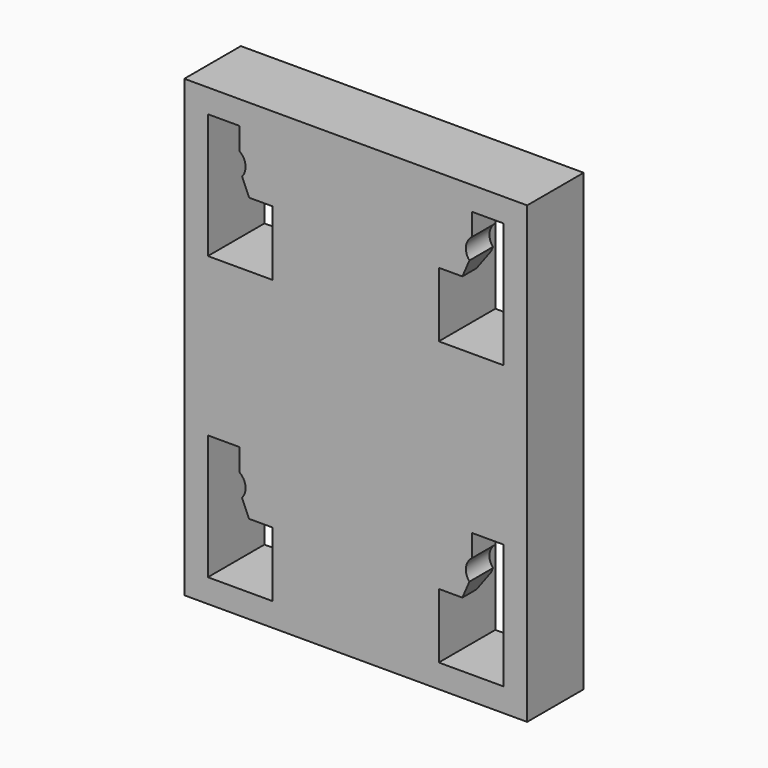
from build123d import *

# Parameters (mm, degrees)
F3_W        = 29.1
F3_H        = 38.6
F4_DEPTH    = 6
F5_T        = 2
F7_DEPTH    = 0.5
F8_T1_DEPTH = 4.571682988
F8_T3_DEPTH = 4.571682988
F9_W        = 10.1
F9_H        = 9.4
F10_DEPTH   = 4


# Not quite as in the source:
# - a fillet or chamfer that OpenCascade refuses, or shapes differently, is made with other operations: its cross-section is extruded or revolved along the edge and cut away or added
# - a feature of the source that left no trace in its solid (it failed there, or was rolled back) is left out
# - a shell that OpenCascade refuses in one call is made with other operations: the cavity is built on its own and cut out


with BuildPart() as f4:
    # F3 (on Front) → F4 (new body)
    with BuildSketch(Plane.XZ):
        Rectangle(F3_W, F3_H)
        with BuildLine():
            Line((-12.55, -17.3), (-12.55, -6.7))
            Line((-12.55, -6.7), (-9.85, -6.7))
            Line((-9.85, -6.7), (-9.85, -8.6))
            ThreePointArc((-9.85, -8.6), (-9.3575419845, -9.4628939105), (-9.65, -10.4124038405))
            Line((-9.65, -10.4124038405), (-9.05, -11.8))
            Line((-9.05, -11.8), (-7.05, -11.8))
            Line((-7.05, -11.8), (-7.05, -17.3))
            Line((-7.05, -17.3), (-12.55, -17.3))
        make_face(mode=Mode.SUBTRACT)
        with BuildLine():
            Line((12.55, -6.7), (12.55, -17.3))
            Line((12.55, -17.3), (7.05, -17.3))
            Line((7.05, -17.3), (7.05, -11.8))
            Line((7.05, -11.8), (9.05, -11.8))
            Line((9.05, -11.8), (9.65, -10.4124038405))
            ThreePointArc((9.65, -10.4124038405), (9.3575419845, -9.4628939105), (9.85, -8.6))
            Line((9.85, -8.6), (9.85, -6.7))
            Line((9.85, -6.7), (12.55, -6.7))
        make_face(mode=Mode.SUBTRACT)
        with BuildLine():
            Line((-12.55, 6.7), (-12.55, 17.3))
            Line((-12.55, 17.3), (-9.85, 17.3))
            Line((-9.85, 17.3), (-9.85, 15.4))
            ThreePointArc((-9.85, 15.4), (-9.3575419845, 14.5371060895), (-9.65, 13.5875961595))
            Line((-9.65, 13.5875961595), (-9.05, 12.2))
            Line((-9.05, 12.2), (-7.05, 12.2))
            Line((-7.05, 12.2), (-7.05, 6.7))
            Line((-7.05, 6.7), (-12.55, 6.7))
        make_face(mode=Mode.SUBTRACT)
        with BuildLine():
            Line((7.05, 6.7), (7.05, 12.2))
            Line((7.05, 12.2), (9.05, 12.2))
            Line((9.05, 12.2), (9.65, 13.5875961595))
            ThreePointArc((9.65, 13.5875961595), (9.3575419845, 14.5371060895), (9.85, 15.4))
            Line((9.85, 15.4), (9.85, 17.3))
            Line((9.85, 17.3), (12.55, 17.3))
            Line((12.55, 17.3), (12.55, 6.7))
            Line((12.55, 6.7), (7.05, 6.7))
        make_face(mode=Mode.SUBTRACT)
    extrude(amount=F4_DEPTH)

    # F5: shell of thickness 2, made by hand


with BuildPart() as f5_core1:
    # F5_t2: copy of F4
    add(f4.part)

    # the walls: a layer under each face that stays
    f5_faces = [f5_core1.faces().sort_by_distance(p)[0] for p in [
        (14.55, -3, 0),
        (0, -3, 19.3),
        (-14.55, -3, 0),
        (0, -3, -19.3),
        (0, -6, 0),
    ]]
    thicken(f5_faces, amount=-F5_T, mode=Mode.SUBTRACT)


with BuildPart() as f4_1:
    add(f4.part)

    # what is left inside the walls is the cavity
    f5_cavity = [f5_core1.part.solids().sort_by_distance(p)[0] for p in [
        (0, -0.02, -5.766667),
    ]]
    add(f5_cavity, mode=Mode.SUBTRACT)

    # F6 (on face) → F7 (join)
    with BuildSketch(Plane(origin=(0, -4, 0), x_dir=(-1, 0, 0), z_dir=(0, 1, 0))):
        with BuildLine():
            Line((-7.05, 17.3), (-9.85, 17.3))
            Line((-9.85, 17.3), (-9.85, 15.4))
            ThreePointArc((-9.85, 15.4), (-9.3575419845, 14.5371060895), (-9.65, 13.5875961595))
            Line((-9.65, 13.5875961595), (-9.05, 12.2))
            Line((-9.05, 12.2), (-7.05, 12.2))
            Line((-7.05, 12.2), (-7.05, 17.3))
        make_face()
        with BuildLine():
            Line((9.85, 17.3), (7.05, 17.3))
            Line((7.05, 17.3), (7.05, 12.2))
            Line((7.05, 12.2), (9.05, 12.2))
            Line((9.05, 12.2), (9.65, 13.5875961595))
            ThreePointArc((9.65, 13.5875961595), (9.3575419845, 14.5371060895), (9.85, 15.4))
            Line((9.85, 15.4), (9.85, 17.3))
        make_face()
        with BuildLine():
            Line((-9.65, -10.4124038405), (-9.05, -11.8))
            Line((-9.05, -11.8), (-7.05, -11.8))
            Line((-7.05, -11.8), (-7.05, -6.7))
            Line((-7.05, -6.7), (-9.85, -6.7))
            Line((-9.85, -6.7), (-9.85, -8.6))
            ThreePointArc((-9.85, -8.6), (-9.3575419845, -9.4628939105), (-9.65, -10.4124038405))
        make_face()
        with BuildLine():
            Line((9.85, -6.7), (7.05, -6.7))
            Line((7.05, -6.7), (7.05, -11.8))
            Line((7.05, -11.8), (9.05, -11.8))
            Line((9.05, -11.8), (9.65, -10.4124038405))
            ThreePointArc((9.65, -10.4124038405), (9.3575419845, -9.4628939105), (9.85, -8.6))
            Line((9.85, -8.6), (9.85, -6.7))
        make_face()
    extrude(amount=F7_DEPTH)

    # F8: chamfer of 1 on 4 edges, made by hand

    # F8_s2 → F8_t1 (cut)
    with BuildSketch(Plane.YZ.offset(7.05)):
        Polygon((-3.5, -10.8), (-4.5, -11.8), (-3.5, -11.8), align=None)
        Polygon((-3.5, 13.2), (-4.5, 12.2), (-3.5, 12.2), align=None)
    extrude(amount=F8_T1_DEPTH, mode=Mode.SUBTRACT)

    # F8_s4 → F8_t3 (cut)
    with BuildSketch(Plane.YZ.offset(-11.621682988)):
        Polygon((-3.5, -10.8), (-4.5, -11.8), (-3.5, -11.8), align=None)
        Polygon((-3.5, 13.2), (-4.5, 12.2), (-3.5, 12.2), align=None)
    extrude(amount=F8_T3_DEPTH, mode=Mode.SUBTRACT)

    # F9 (on face) → F10 (join, through all)
    with BuildSketch(Plane(origin=(0, -4, 0), x_dir=(-1, 0, 0), z_dir=(0, 1, 0))):
        Polygon((7.05, -17.3), (7.05, -11.3), (7.05, -6.7), (9.85, -6.7), (12.55, -6.7), (12.55, -4.7), (7.05, -4.7), (7.05, 4.7), (12.55, 4.7), (12.55, 6.7), (7.05, 6.7), (7.05, 12.7), (7.05, 17.3), (5.05, 17.3), (5.05, 6.7), (-5.05, 6.7), (-5.05, 17.3), (-7.05, 17.3), (-7.05, 12.7), (-7.05, 6.7), (-12.55, 6.7), (-12.55, 4.7), (-7.05, 4.7), (-7.05, -4.7), (-12.55, -4.7), (-12.55, -6.7), (-9.85, -6.7), (-7.05, -6.7), (-7.05, -11.3), (-7.05, -17.3), (-5.05, -17.3), (-5.05, -6.7), (5.05, -6.7), (5.05, -17.3), align=None)
        Rectangle(F9_W, F9_H, mode=Mode.SUBTRACT)
    extrude(amount=F10_DEPTH)


solid = f4_1.part
